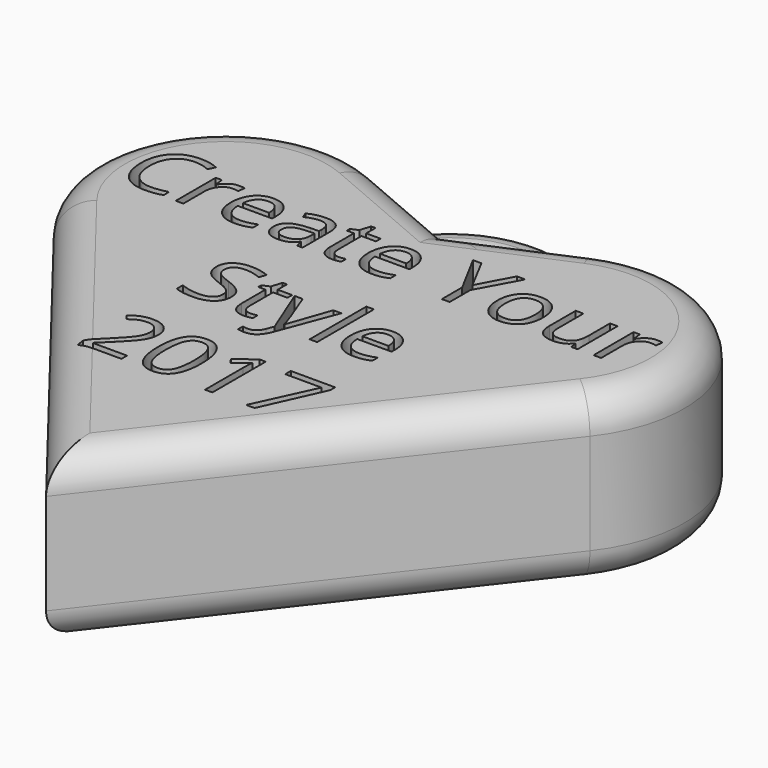
from build123d import *

# Parameters (mm, degrees)
F1_DEPTH     = 5
F2_R         = 8
F3_R         = 7
F3_R_2       = 4
F4_DEPTH     = 1.5
F5_R         = 1.49999
F6_TEXT_SIZE = 5.5555555556
F7_DEPTH     = 3
F8_T1_DEPTH  = 30.9929287056
F8_T3_DEPTH  = 30.9929287056
F8_T6_ANGLE  = 151.0735741647
F8_T10_DEPTH = 12.0630229799
F8_T13_ANGLE = 151.0735741647
F8_T17_DEPTH = 12.0630229799
F8_T20_ANGLE = 151.0735741647
F8_T24_DEPTH = 12.0630229799
F8_T29_DEPTH = 12.0630229799
F8_T32_ANGLE = 151.0735741647
F8_T37_DEPTH = 12.0630229799
F8_T41_DEPTH = 12.0630229799
F8_T48_DEPTH = 12.0630229799
F8_T52_DEPTH = 12.0630229799


# Not quite as in the source:
# - a fillet or chamfer that OpenCascade refuses, or shapes differently, is made with other operations: its cross-section is extruded or revolved along the edge and cut away or added
# - a fillet or chamfer is up to 0.001 mm smaller than in the source, because OpenCascade refuses the exact size
# - Text() gives the source's letters only with a copy of the font that has no kerning and outlines rounded to 1/6400 em; it was checked with that copy


with BuildPart() as f1:
    # F0 (on Top) → F1 (new body, symmetric)
    with BuildSketch(Plane.XY):
        Polygon((-35, 45), (0, 0), (35, 45), (0, 30), align=None)
    extrude(amount=F1_DEPTH, both=True)

    # F2
    f2_edges = [f1.edges().sort_by_distance(p)[0] for p in [
        (-35, 45, 0),
        (35, 45, 0),
    ]]
    fillet(f2_edges, radius=F2_R)

    # F3 (on Top) → F4 (join, symmetric)
    with BuildSketch(Plane.XY):
        with Locations((0, 30)):
            Circle(F3_R)
        with Locations((0, 30)):
            Circle(F3_R_2, mode=Mode.SUBTRACT)
    extrude(amount=F4_DEPTH, both=True)

    # F5 (radius 1.5 in the source; OpenCascade refuses exactly that, so slightly less here)
    f5_edges = [f1.edges().sort_by_distance(p)[0] for p in [
        (0, 37, 1.5),
        (0, 34, 1.5),
        (0, 34, -1.5),
        (0, 37, -1.5),
    ]]
    fillet(f5_edges, radius=F5_R)

    # F6 (on face) → F7 (cut)
    with BuildSketch(Plane.XY.offset(5)):
        with Locations((-15.4639756944, 24)):
            Text('Create Your', F6_TEXT_SIZE, font='Open Sans', text_align=(TextAlign.LEFT, TextAlign.BOTTOM))
        with Locations((-6.2009548611, 17)):
            Text('Style', F6_TEXT_SIZE, font='Open Sans', text_align=(TextAlign.LEFT, TextAlign.BOTTOM))
        with Locations((-6.3914930556, 10)):
            Text('2017', F6_TEXT_SIZE, font='Open Sans', text_align=(TextAlign.LEFT, TextAlign.BOTTOM))
    extrude(amount=-F7_DEPTH, mode=Mode.SUBTRACT)

    # F8: fillet of radius 2 on 12 edges, made by hand

    # F8_s2 → F8_t1 (cut)
    with BuildSketch(Plane(origin=(-15.9581145965, 20.5175759098, 0), x_dir=(0, 0, 1), z_dir=(0.6139406135, -0.7893522174, 0))):
        with BuildLine():
            ThreePointArc((-5, -2), (-4.4142135624, -0.5857864376), (-3, 0))
            Line((-3, 0), (-5, 0))
            Line((-5, 0), (-5, -2))
        make_face()
        with BuildLine():
            ThreePointArc((5, -2), (4.4142135624, -0.5857864376), (3, 0))
            Line((3, 0), (5, 0))
            Line((5, 0), (5, -2))
        make_face()
    extrude(amount=F8_T1_DEPTH, mode=Mode.SUBTRACT)

    # F8_s4 → F8_t3 (cut)
    with BuildSketch(Plane(origin=(-3.0697030676, -3.9467610869, 0), x_dir=(0, 0, 1), z_dir=(0.6139406135, 0.7893522174, 0))):
        with BuildLine():
            ThreePointArc((-5, -2), (-4.4142135624, -0.5857864376), (-3, 0))
            Line((-3, 0), (-5, 0))
            Line((-5, 0), (-5, -2))
        make_face()
        with BuildLine():
            ThreePointArc((5, -2), (4.4142135624, -0.5857864376), (3, 0))
            Line((3, 0), (5, 0))
            Line((5, 0), (5, -2))
        make_face()
    extrude(amount=F8_T3_DEPTH, mode=Mode.SUBTRACT)

    # F8_s5 → F8_t6 (revolve, cut)
    with BuildSketch(Plane(origin=(-15.9581145965, 20.5175759098, 0), x_dir=(0, 0, 1), z_dir=(0.6139406135, -0.7893522174, 0))):
        with BuildLine():
            ThreePointArc((-5, -2), (-4.4142135624, -0.5857864376), (-3, 0))
            Line((-3, 0), (-5, 0))
            Line((-5, 0), (-5, -2))
        make_face()
    revolve(axis=Axis((-9.6432968575, 25.429100818, -5), (0, 0, -1)), revolution_arc=F8_T6_ANGLE, mode=Mode.SUBTRACT)


with BuildPart() as f8_tool8:
    # F8_s9 → F8_t10 (new body)
    with BuildSketch(Plane(origin=(-6.2663438154, 2.6855759209, 0), x_dir=(0, 0, 1), z_dir=(-0.91914503, 0.3939192986, 0))):
        with BuildLine():
            ThreePointArc((-3, 27.5743509005), (-4.4142135624, 26.9885644629), (-5, 25.5743509005))
            Line((-5, 25.5743509005), (-5, 27.5743509005))
            Line((-5, 27.5743509005), (-3, 27.5743509005))
        make_face()
    extrude(amount=F8_T10_DEPTH)

    split(bisect_by=Plane(origin=(-10.8620689655, 25.3448275862, 0), x_dir=(0, 0, 1), z_dir=(-0.3939192986, 0.91914503, 0)), keep=Keep.TOP)


with BuildPart() as f1_1:
    add(f1.part)

    # F8_t7: cut F8_tool8
    add(f8_tool8.part, mode=Mode.SUBTRACT)

    # F8_s12 → F8_t13 (revolve, cut)
    with BuildSketch(Plane(origin=(17.3540114344, 7.4374334719, 0), x_dir=(0, 0, 1), z_dir=(-0.91914503, -0.3939192986, 0))):
        with BuildLine():
            ThreePointArc((-5, 25.5743509005), (-4.4142135624, 26.9885644629), (-3, 27.5743509005))
            Line((-3, 27.5743509005), (-5, 27.5743509005))
            Line((-5, 27.5743509005), (-5, 25.5743509005))
        make_face()
    revolve(axis=Axis((9.6432968575, 25.429100818, -5), (0, 0, -1)), revolution_arc=F8_T13_ANGLE, mode=Mode.SUBTRACT)


with BuildPart() as f8_tool15:
    # F8_s16 → F8_t17 (new body)
    with BuildSketch(Plane(origin=(17.3540114344, 7.4374334719, 0), x_dir=(0, 0, 1), z_dir=(-0.91914503, -0.3939192986, 0))):
        with BuildLine():
            ThreePointArc((-5, 25.5743509005), (-4.4142135624, 26.9885644629), (-3, 27.5743509005))
            Line((-3, 27.5743509005), (-5, 27.5743509005))
            Line((-5, 27.5743509005), (-5, 25.5743509005))
        make_face()
    extrude(amount=F8_T17_DEPTH)

    split(bisect_by=Plane(origin=(10.8620689655, 25.3448275862, 0), x_dir=(0, 0, 1), z_dir=(0.3939192986, 0.91914503, 0)), keep=Keep.TOP)


with BuildPart() as f1_2:
    add(f1_1.part)

    # F8_t14: cut F8_tool15
    add(f8_tool15.part, mode=Mode.SUBTRACT)

    # F8_s19 → F8_t20 (revolve, cut)
    with BuildSketch(Plane(origin=(-15.9581145965, 20.5175759098, 0), x_dir=(0, 0, 1), z_dir=(0.6139406135, -0.7893522174, 0))):
        with BuildLine():
            ThreePointArc((3, 0), (4.4142135624, -0.5857864376), (5, -2))
            Line((5, -2), (5, 0))
            Line((5, 0), (3, 0))
        make_face()
    revolve(axis=Axis((-9.6432968575, 25.429100818, 5), (0, 0, -1)), revolution_arc=F8_T20_ANGLE, mode=Mode.SUBTRACT)


with BuildPart() as f8_tool22:
    # F8_s23 → F8_t24 (new body)
    with BuildSketch(Plane(origin=(-6.2663438154, 2.6855759209, 0), x_dir=(0, 0, 1), z_dir=(-0.91914503, 0.3939192986, 0))):
        with BuildLine():
            ThreePointArc((3, 27.5743509005), (4.4142135624, 26.9885644629), (5, 25.5743509005))
            Line((5, 25.5743509005), (5, 27.5743509005))
            Line((5, 27.5743509005), (3, 27.5743509005))
        make_face()
    extrude(amount=F8_T24_DEPTH)

    split(bisect_by=Plane(origin=(-10.8620689655, 25.3448275862, 0), x_dir=(0, 0, 1), z_dir=(-0.3939192986, 0.91914503, 0)), keep=Keep.TOP)


with BuildPart() as f1_3:
    add(f1_2.part)

    # F8_t21: cut F8_tool22
    add(f8_tool22.part, mode=Mode.SUBTRACT)


with BuildPart() as f8_tool27:
    # F8_s28 → F8_t29 (new body)
    with BuildSketch(Plane(origin=(17.3540114344, 7.4374334719, 0), x_dir=(0, 0, 1), z_dir=(-0.91914503, -0.3939192986, 0))):
        with BuildLine():
            ThreePointArc((3, 27.5743509005), (4.4142135624, 26.9885644629), (5, 25.5743509005))
            Line((5, 25.5743509005), (5, 27.5743509005))
            Line((5, 27.5743509005), (3, 27.5743509005))
        make_face()
    extrude(amount=F8_T29_DEPTH)

    split(bisect_by=Plane(origin=(10.8620689655, 25.3448275862, 0), x_dir=(0, 0, 1), z_dir=(0.3939192986, 0.91914503, 0)), keep=Keep.TOP)


with BuildPart() as f1_4:
    add(f1_3.part)

    # F8_t26: cut F8_tool27
    add(f8_tool27.part, mode=Mode.SUBTRACT)

    # F8_s31 → F8_t32 (revolve, cut)
    with BuildSketch(Plane(origin=(17.3540114344, 7.4374334719, 0), x_dir=(0, 0, 1), z_dir=(-0.91914503, -0.3939192986, 0))):
        with BuildLine():
            ThreePointArc((5, 25.5743509005), (4.4142135624, 26.9885644629), (3, 27.5743509005))
            Line((3, 27.5743509005), (5, 27.5743509005))
            Line((5, 27.5743509005), (5, 25.5743509005))
        make_face()
    revolve(axis=Axis((9.6432968575, 25.429100818, 5), (0, 0, -1)), revolution_arc=F8_T32_ANGLE, mode=Mode.SUBTRACT)


with BuildPart() as f8_tool35:
    # F8_s36 → F8_t37 (new body)
    with BuildSketch(Plane(origin=(-6.2663438154, 2.6855759209, 0), x_dir=(0, 0, 1), z_dir=(-0.91914503, 0.3939192986, 0))):
        with BuildLine():
            ThreePointArc((-3, 27.5743509005), (-4.4142135624, 26.9885644629), (-5, 25.5743509005))
            Line((-5, 25.5743509005), (-5, 27.5743509005))
            Line((-5, 27.5743509005), (-3, 27.5743509005))
        make_face()
    extrude(amount=F8_T37_DEPTH)

    split(bisect_by=Plane(origin=(-10.8620689655, 25.3448275862, 0), x_dir=(0, 0, 1), z_dir=(0.3939192986, -0.91914503, 0)), keep=Keep.TOP)


with BuildPart() as f8_tool39:
    # F8_s40 → F8_t41 (new body)
    with BuildSketch(Plane(origin=(17.3540114344, 7.4374334719, 0), x_dir=(0, 0, 1), z_dir=(-0.91914503, -0.3939192986, 0))):
        with BuildLine():
            ThreePointArc((-5, 25.5743509005), (-4.4142135624, 26.9885644629), (-3, 27.5743509005))
            Line((-3, 27.5743509005), (-5, 27.5743509005))
            Line((-5, 27.5743509005), (-5, 25.5743509005))
        make_face()
    extrude(amount=F8_T41_DEPTH)

    split(bisect_by=Plane(origin=(10.8620689655, 25.3448275862, 0), x_dir=(0, 0, 1), z_dir=(-0.3939192986, -0.91914503, 0)), keep=Keep.TOP)


with BuildPart() as f8_tool35_1:
    add(f8_tool35.part)

    # F8_t43: intersect F8_tool39
    add(f8_tool39.part, mode=Mode.INTERSECT)


with BuildPart() as f1_5:
    add(f1_4.part)

    # F8_t33: cut F8_tool35
    add(f8_tool35_1.part, mode=Mode.SUBTRACT)


with BuildPart() as f8_tool46:
    # F8_s47 → F8_t48 (new body)
    with BuildSketch(Plane(origin=(-6.2663438154, 2.6855759209, 0), x_dir=(0, 0, 1), z_dir=(-0.91914503, 0.3939192986, 0))):
        with BuildLine():
            ThreePointArc((3, 27.5743509005), (4.4142135624, 26.9885644629), (5, 25.5743509005))
            Line((5, 25.5743509005), (5, 27.5743509005))
            Line((5, 27.5743509005), (3, 27.5743509005))
        make_face()
    extrude(amount=F8_T48_DEPTH)

    split(bisect_by=Plane(origin=(-10.8620689655, 25.3448275862, 0), x_dir=(0, 0, 1), z_dir=(0.3939192986, -0.91914503, 0)), keep=Keep.TOP)


with BuildPart() as f8_tool50:
    # F8_s51 → F8_t52 (new body)
    with BuildSketch(Plane(origin=(17.3540114344, 7.4374334719, 0), x_dir=(0, 0, 1), z_dir=(-0.91914503, -0.3939192986, 0))):
        with BuildLine():
            ThreePointArc((3, 27.5743509005), (4.4142135624, 26.9885644629), (5, 25.5743509005))
            Line((5, 25.5743509005), (5, 27.5743509005))
            Line((5, 27.5743509005), (3, 27.5743509005))
        make_face()
    extrude(amount=F8_T52_DEPTH)

    split(bisect_by=Plane(origin=(10.8620689655, 25.3448275862, 0), x_dir=(0, 0, 1), z_dir=(-0.3939192986, -0.91914503, 0)), keep=Keep.TOP)


with BuildPart() as f8_tool46_1:
    add(f8_tool46.part)

    # F8_t54: intersect F8_tool50
    add(f8_tool50.part, mode=Mode.INTERSECT)


with BuildPart() as f1_6:
    add(f1_5.part)

    # F8_t44: cut F8_tool46
    add(f8_tool46_1.part, mode=Mode.SUBTRACT)


solid = f1_6.part
